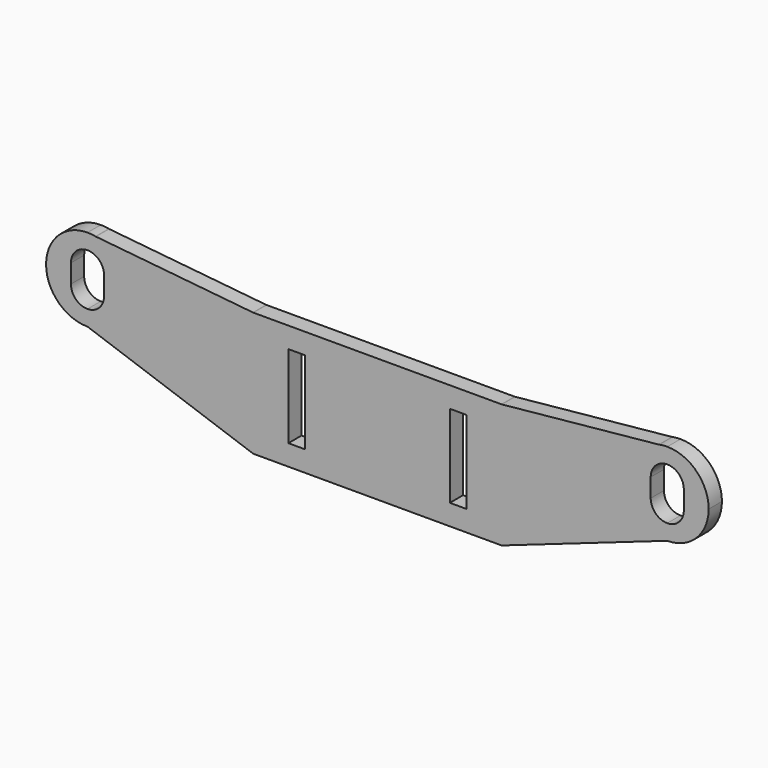
from build123d import *

# Parameters (mm, degrees)
F0_W        = 120
F0_H        = 60
F0_W_2      = 8
F0_H_2      = 40
F1_DEPTH    = 8
F2_T1_DEPTH = 8
F2_T3_DEPTH = 9.6994572863


# Not quite as in the source:
# - a fillet or chamfer that OpenCascade refuses, or shapes differently, is made with other operations: its cross-section is extruded or revolved along the edge and cut away or added


with BuildPart() as f1:
    # F0 (on Front) → F1 (new body)
    with BuildSketch(Plane.XZ):
        with Locations((-60, -30)):
            Rectangle(F0_W, F0_H)
        with Locations((-99, -30)):
            Rectangle(F0_W_2, F0_H_2, mode=Mode.SUBTRACT)
        with Locations((-21, -30)):
            Rectangle(F0_W_2, F0_H_2, mode=Mode.SUBTRACT)
        with BuildLine():
            Line((76.0396039604, 7.603960396), (0, 0))
            Line((0, 0), (0, -60))
            Line((0, -60), (80, -32))
            ThreePointArc((80, -32), (60.0992561958, -13.9900743804), (76.0396039604, 7.603960396))
        make_face()
        with BuildLine():
            Line((-120, -60), (-120, 0))
            Line((-120, 0), (-196.0396039604, 7.603960396))
            ThreePointArc((-196.0396039604, 7.603960396), (-184.5208540159, 0.6647558051), (-180, -12))
            ThreePointArc((-180, -12), (-185.8578643763, -26.1421356237), (-200, -32))
            Line((-200, -32), (-120, -60))
        make_face()
        with BuildLine():
            ThreePointArc((80, 8), (78.0099256196, 7.9007438042), (76.0396039604, 7.603960396))
            Line((76.0396039604, 7.603960396), (80, 8))
        make_face()
        with BuildLine():
            Line((80, 8), (76.0396039604, 7.603960396))
            ThreePointArc((76.0396039604, 7.603960396), (60.0992561958, -13.9900743804), (80, -32))
            Line((80, -32), (80, -24.5))
            ThreePointArc((80, -24.5), (74.3431457505, -22.1568542495), (72, -16.5))
            Line((72, -16.5), (72, -7.5))
            ThreePointArc((72, -7.5), (74.3431457505, -1.8431457505), (80, 0.5))
            Line((80, 0.5), (80, 8))
        make_face()
        with BuildLine():
            ThreePointArc((-180, -12), (-184.5208540159, 0.6647558051), (-196.0396039604, 7.603960396))
            Line((-196.0396039604, 7.603960396), (-200, 8))
            Line((-200, 8), (-200, 0.5))
            ThreePointArc((-200, 0.5), (-194.3431457505, -1.8431457505), (-192, -7.5))
            Line((-192, -7.5), (-192, -16.5))
            ThreePointArc((-192, -16.5), (-194.3431457505, -22.1568542495), (-200, -24.5))
            Line((-200, -24.5), (-200, -32))
            ThreePointArc((-200, -32), (-185.8578643763, -26.1421356237), (-180, -12))
        make_face()
        with BuildLine():
            Line((-200, 8), (-196.0396039604, 7.603960396))
            ThreePointArc((-196.0396039604, 7.603960396), (-198.0099256196, 7.9007438042), (-200, 8))
        make_face()
        with BuildLine():
            Line((80, -24.5), (80, -32))
            ThreePointArc((80, -32), (94.1421356237, -26.1421356237), (100, -12))
            ThreePointArc((100, -12), (94.1421356237, 2.1421356237), (80, 8))
            Line((80, 8), (80, 0.5))
            ThreePointArc((80, 0.5), (85.6568542495, -1.8431457505), (88, -7.5))
            Line((88, -7.5), (88, -16.5))
            ThreePointArc((88, -16.5), (85.6568542495, -22.1568542495), (80, -24.5))
        make_face()
        with BuildLine():
            ThreePointArc((-200, 8), (-220, -12), (-200, -32))
            Line((-200, -32), (-200, -24.5))
            ThreePointArc((-200, -24.5), (-205.6568542495, -22.1568542495), (-208, -16.5))
            Line((-208, -16.5), (-208, -7.5))
            ThreePointArc((-208, -7.5), (-205.6568542495, -1.8431457505), (-200, 0.5))
            Line((-200, 0.5), (-200, 8))
        make_face()
    extrude(amount=F1_DEPTH)

    # F2: fillet of radius 2 on 7 edges, made by hand

    # F2_s2 → F2_t1 (join)
    with BuildSketch(Plane.XZ):
        with BuildLine():
            ThreePointArc((-119.9002487578, 0), (-119.9998761615, 0.0024829462), (-120.0992561958, 0.0099256196))
            Line((-120.0992561958, 0.0099256196), (-120, 0))
            Line((-120, 0), (-119.9002487578, 0))
        make_face()
        with BuildLine():
            ThreePointArc((-0.0997512422, 0), (-0.0001238385, 0.0024829462), (0.0992561958, 0.0099256196))
            Line((0.0992561958, 0.0099256196), (0, 0))
            Line((0, 0), (-0.0997512422, 0))
        make_face()
        with BuildLine():
            ThreePointArc((-200.316131174, -31.9975013709), (-199.9970841579, -32.0282320894), (-199.687043442, -32.1095347953))
            Line((-199.687043442, -32.1095347953), (-200, -32))
            ThreePointArc((-200, -32), (-200.1580705241, -31.999375333), (-200.316131174, -31.9975013709))
        make_face()
        with BuildLine():
            ThreePointArc((79.687043442, -32.1095347953), (79.997084158, -32.0282320894), (80.316131174, -31.9975013709))
            ThreePointArc((80.316131174, -31.9975013709), (80.1580705241, -31.999375333), (80, -32))
            Line((80, -32), (79.687043442, -32.1095347953))
        make_face()
        with BuildLine():
            ThreePointArc((76.1306459256, 7.6221328873), (76.0370129468, 7.6059696483), (75.9427179562, 7.5942717956))
            Line((75.9427179562, 7.5942717956), (76.0396039604, 7.603960396))
            ThreePointArc((76.0396039604, 7.603960396), (76.0851143987, 7.6130994677), (76.1306459256, 7.6221328873))
        make_face()
        with BuildLine():
            ThreePointArc((-195.9427179562, 7.5942717956), (-196.0370129468, 7.6059696483), (-196.1306459256, 7.6221328873))
            ThreePointArc((-196.1306459256, 7.6221328873), (-196.0851143987, 7.6130994677), (-196.0396039604, 7.603960396))
            Line((-196.0396039604, 7.603960396), (-195.9427179562, 7.5942717956))
        make_face()
    extrude(amount=F2_T1_DEPTH)

    # F2_s4 → F2_t3 (cut)
    with BuildSketch(Plane.XZ.offset(-0.8497286432)):
        with BuildLine():
            ThreePointArc((-120.3208093922, -59.8877167127), (-119.9951955274, -59.9717293711), (-119.6601085427, -60))
            Line((-119.6601085427, -60), (-120, -60))
            Line((-120, -60), (-120.3208093922, -59.8877167127))
        make_face()
    extrude(amount=F2_T3_DEPTH, mode=Mode.SUBTRACT)


solid = f1.part
